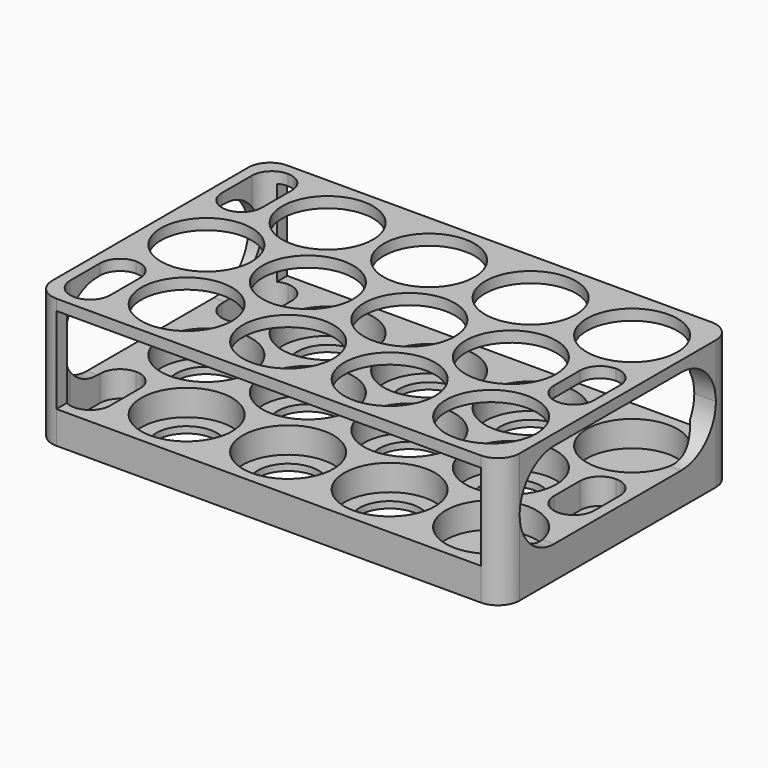
from build123d import *

# Parameters (mm, degrees)
F1_DEPTH = 137.4775
F2_W     = 124.7775
F2_H     = 25.4
F2_W_2   = 12.7
F2_H_2   = 3.175
F2_W_3   = 99.3775
F3_DEPTH = 84.837
F4_R     = 13.335
F5_DEPTH = 36.195
F6_R     = 6.34999
F7_R     = 8.89
F8_DEPTH = 12.7
F9_R     = 6.35


# Not quite as in the source:
# - a fillet or chamfer is up to 0.001 mm smaller than in the source, because OpenCascade refuses the exact size
# - a feature names something its author has since deleted; it is built from what else it names


with BuildPart() as f1:
    # F0 (on Right) → F1 (new body)
    with BuildSketch(Plane.YZ):
        Polygon((42.418, -17.4625), (42.418, 20.6375), (-42.418, 20.6375), (-42.418, -17.4625), (-36.068, -17.4625), (-28.448, -20.6375), (-22.098, -20.6375), (-14.478, -17.4625), (14.478, -17.4625), (22.098, -20.6375), (28.448, -20.6375), (36.068, -17.4625), align=None)
        with BuildLine():
            Line((-23.368, 17.4625), (23.368, 17.4625))
            ThreePointArc((23.368, 17.4625), (32.3482561211, 13.7427561211), (36.068, 4.7625))
            ThreePointArc((36.068, 4.7625), (32.3482561211, -4.2177561211), (23.368, -7.9375))
            Line((23.368, -7.9375), (-23.368, -7.9375))
            ThreePointArc((-23.368, -7.9375), (-32.3482561211, -4.2177561211), (-36.068, 4.7625))
            ThreePointArc((-36.068, 4.7625), (-32.3482561211, 13.7427561211), (-23.368, 17.4625))
        make_face(mode=Mode.SUBTRACT)
    extrude(amount=F1_DEPTH)

    # F2 (on face) → F3 (cut, through all)
    with BuildSketch(Plane(origin=(0, 42.418, 0), x_dir=(-1, 0, 0), z_dir=(0, 1, 0))):
        with Locations((-68.73875, 4.7625)):
            Rectangle(F2_W, F2_H)
        with Locations((-131.1275, -19.05)):
            Rectangle(F2_W_2, F2_H_2)
        with Locations((-68.73875, -19.05)):
            Rectangle(F2_W_3, F2_H_2)
        with Locations((-6.35, -19.05)):
            Rectangle(F2_W_2, F2_H_2)
    extrude(amount=-F3_DEPTH, mode=Mode.SUBTRACT)

    # F4 (on face) → F5 (cut)
    with BuildSketch(Plane.XY.offset(20.6375)):
        with Locations((16.51, 0)):
            Circle(F4_R)
        with Locations((46.355, 0)):
            Circle(F4_R)
        with Locations((76.2, 0)):
            Circle(F4_R)
        with Locations((106.045, 0)):
            Circle(F4_R)
        with Locations((120.9675, -25.908)):
            Circle(F4_R)
        with Locations((91.1225, -25.908)):
            Circle(F4_R)
        with Locations((61.2775, -25.908)):
            Circle(F4_R)
        with Locations((31.4325, -25.908)):
            Circle(F4_R)
        with Locations((31.4325, 25.908)):
            Circle(F4_R)
        with Locations((61.2775, 25.908)):
            Circle(F4_R)
        with Locations((91.1225, 25.908)):
            Circle(F4_R)
        with Locations((120.9675, 25.908)):
            Circle(F4_R)
        with BuildLine():
            ThreePointArc((9.04875, -16.51), (4.895381544, -18.230381544), (3.175, -22.38375))
            Line((3.175, -22.38375), (3.175, -33.36925))
            ThreePointArc((3.175, -33.36925), (4.895381544, -37.522618456), (9.04875, -39.243))
            ThreePointArc((9.04875, -39.243), (13.202118456, -37.522618456), (14.9225, -33.36925))
            Line((14.9225, -33.36925), (14.9225, -22.38375))
            ThreePointArc((14.9225, -22.38375), (13.202118456, -18.230381544), (9.04875, -16.51))
        make_face()
        with BuildLine():
            ThreePointArc((9.04875, 16.51), (13.202118456, 18.230381544), (14.9225, 22.38375))
            Line((14.9225, 22.38375), (14.9225, 33.36925))
            ThreePointArc((14.9225, 33.36925), (13.202118456, 37.522618456), (9.04875, 39.243))
            ThreePointArc((9.04875, 39.243), (4.895381544, 37.522618456), (3.175, 33.36925))
            Line((3.175, 33.36925), (3.175, 22.38375))
            ThreePointArc((3.175, 22.38375), (4.895381544, 18.230381544), (9.04875, 16.51))
        make_face()
        with BuildLine():
            Line((134.3025, -4.79425), (134.3025, 4.79425))
            ThreePointArc((134.3025, 4.79425), (132.582118456, 8.947618456), (128.42875, 10.668))
            ThreePointArc((128.42875, 10.668), (124.275381544, 8.947618456), (122.555, 4.79425))
            Line((122.555, 4.79425), (122.555, -4.79425))
            ThreePointArc((122.555, -4.79425), (124.275381544, -8.947618456), (128.42875, -10.668))
            ThreePointArc((128.42875, -10.668), (132.582118456, -8.947618456), (134.3025, -4.79425))
        make_face()
    extrude(amount=-F5_DEPTH, mode=Mode.SUBTRACT)

    # F6 (radius 6.35 in the source; OpenCascade refuses exactly that, so slightly less here)
    f6_edges = [f1.edges().sort_by_distance(p)[0] for p in [
        (0, 42.418, 1.5875),
        (0, -42.418, 1.5875),
        (137.4775, -42.418, 1.5875),
        (137.4775, 42.418, 1.5875),
    ]]
    fillet(f6_edges, radius=F6_R)

    # F7 (on face) → F8 (cut, symmetric)
    with BuildSketch(Plane(origin=(0, 0, -17.4625), x_dir=(1, 0, 0), z_dir=(0, 0, -1))):
        with Locations((16.51, 0)):
            Circle(F7_R)
        with Locations((46.355, 0)):
            Circle(F7_R)
        with Locations((76.2, 0)):
            Circle(F7_R)
        with Locations((106.045, 0)):
            Circle(F7_R)
        with Locations((31.4325, 25.908)):
            Circle(F7_R)
        with Locations((61.2775, 25.908)):
            Circle(F7_R)
        with Locations((91.1225, 25.908)):
            Circle(F7_R)
        with Locations((91.1225, -25.908)):
            Circle(F7_R)
        with Locations((61.2775, -25.908)):
            Circle(F7_R)
        with Locations((31.4325, -25.908)):
            Circle(F7_R)
    extrude(amount=F8_DEPTH, both=True, mode=Mode.SUBTRACT)

    # F9
    f9_edges = [f1.edges().sort_by_distance(p)[0] for p in [
        (121.6025, 28.448, -20.6375),
        (121.6025, 22.098, -20.6375),
        (121.6025, -22.098, -20.6375),
        (121.6025, -28.448, -20.6375),
        (15.875, 28.448, -20.6375),
        (15.875, 22.098, -20.6375),
        (15.875, -22.098, -20.6375),
        (15.875, -28.448, -20.6375),
    ]]
    fillet(f9_edges, radius=F9_R)


solid = f1.part
